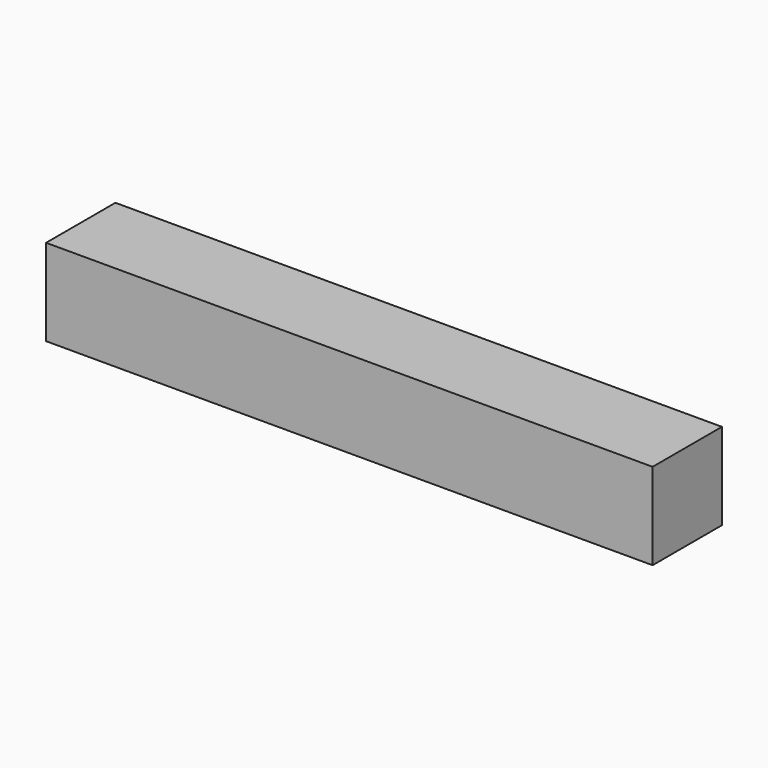
from build123d import *

# Parameters (mm, degrees)
F0_W     = 177.8
F0_H     = 25.4
F1_DEPTH = 25.4


# Not quite as in the source:
# - a feature names something its author has since deleted; it is built from what else it names


with BuildPart() as f1:
    # F0 (on Front) → F1 (new body)
    with BuildSketch(Plane.XZ):
        with Locations((88.9, 12.7)):
            Rectangle(F0_W, F0_H)
    extrude(amount=F1_DEPTH)


solid = f1.part
